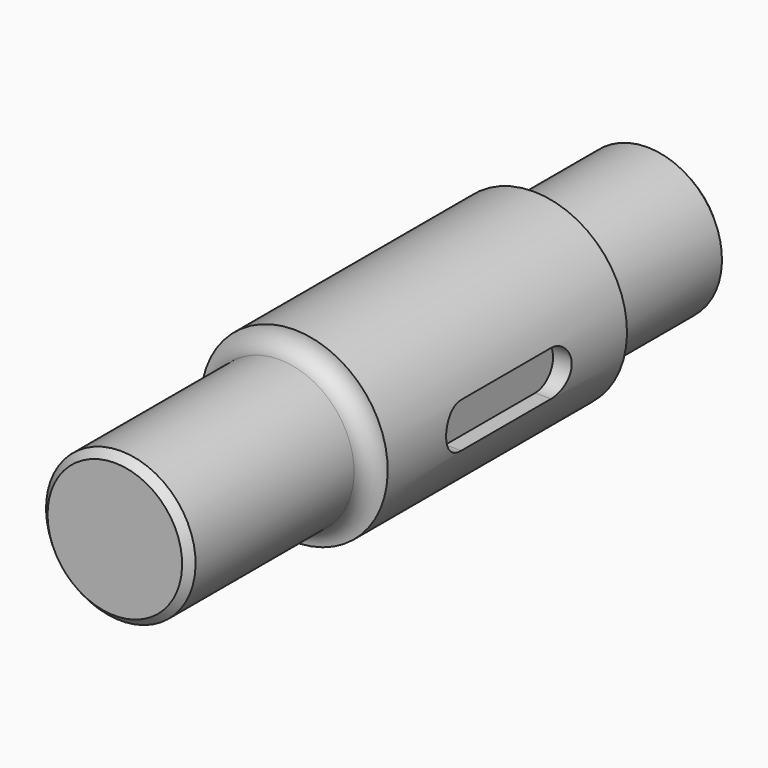
from build123d import *

# Parameters (mm, degrees)
F4_SIZE  = 2
F5_R     = 4.99999
F6_DEPTH = 5


# Not quite as in the source:
# - a fillet or chamfer is up to 0.001 mm smaller than in the source, because OpenCascade refuses the exact size


with BuildPart() as f1:
    # F0 (on Right) → F1 (revolve)
    with BuildSketch(Plane.YZ):
        Polygon((8.0283725262, 25), (0, 25), (-71.9716274738, 25), (-71.9716274738, 20), (-131.9716274738, 20), (-131.9716274738, 0), (48.0283725262, 0), (48.0283725262, 20), (8.0283725262, 20), align=None)
    revolve(axis=Axis((0, -30.3001217544, 0), (0, 1, 0)))

    # F4
    f4_edges = [f1.edges().sort_by_distance(p)[0] for p in [
        (0, -131.971627, -20),
        (0, 48.028373, -20),
    ]]
    chamfer(f4_edges, length=F4_SIZE)

    # F5 (radius 5 in the source; OpenCascade refuses exactly that, so slightly less here)
    f5_edges = [f1.edges().sort_by_distance(p)[0] for p in [
        (0, -71.971627, -20),
        (0, 8.028373, -20),
    ]]
    fillet(f5_edges, radius=F5_R)

    # F3 (on offset) → F6 (cut)
    with BuildSketch(Plane.YZ.offset(25)):
        with BuildLine():
            Line((-16.4436194198, 6), (-46.4436194198, 6))
            ThreePointArc((-46.4436194198, 6), (-52.4436194198, 0), (-46.4436194198, -6))
            Line((-46.4436194198, -6), (-16.4436194198, -6))
            ThreePointArc((-16.4436194198, -6), (-10.4436194198, 0), (-16.4436194198, 6))
        make_face()
    extrude(amount=-F6_DEPTH, mode=Mode.SUBTRACT)


solid = f1.part
